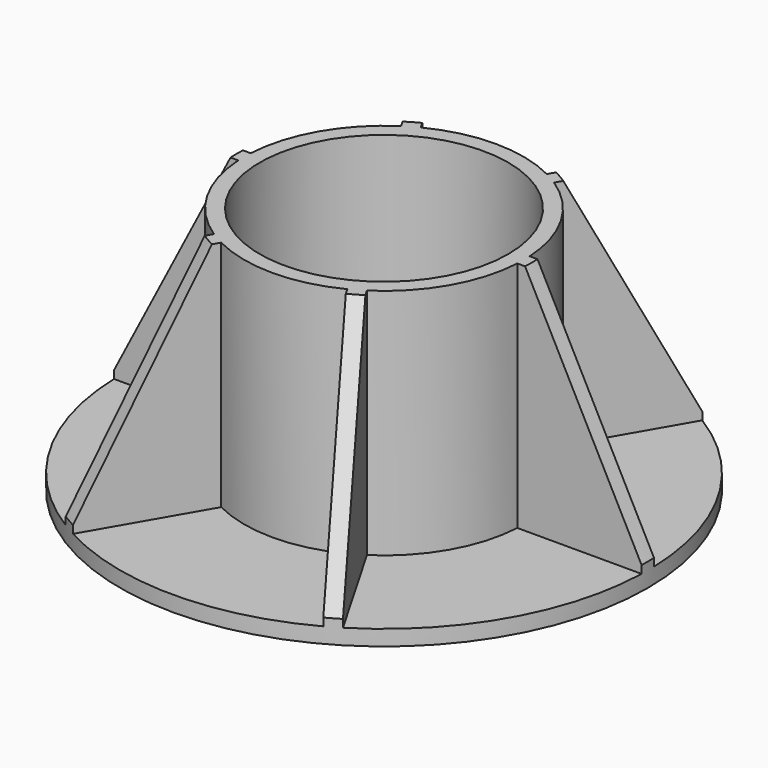
from build123d import *

# Parameters (mm, degrees)
F0_R            = 28.575
F0_R_2          = 25.4
F1_DEPTH        = 12.7
F2_R            = 53.975
F2_R_2          = 25.4
F3_DEPTH        = 50.8
F6_DEPTH        = 47.625
F6_COPIES_COUNT = 6


# Not quite as in the source:
# - a pattern or mirror of a feature is missing from the dataset's text; its kind, count and spacing are read off the source's solid


with BuildPart() as f1:
    # F0 (on Top) → F1 (new body)
    with BuildSketch(Plane.XY):
        Circle(F0_R)
        Circle(F0_R_2, mode=Mode.SUBTRACT)
    extrude(amount=F1_DEPTH)

    # F2 (on face) → F3 (join)
    with BuildSketch(Plane.XY.offset(12.7)):
        Circle(F2_R)
        Circle(F2_R_2, mode=Mode.SUBTRACT)
    extrude(amount=F3_DEPTH)

    # F5 (on face) → F6 (cut, through all)
    with BuildSketch(Plane.XY.offset(63.5)):
        with BuildLine():
            ThreePointArc((-15.6402496783, -23.9147070858), (-24.7466759131, -14.2875), (-28.5308686995, -1.5875))
            Line((-28.5308686995, -1.5875), (-53.9516493608, -1.5875))
            ThreePointArc((-53.9516493608, -1.5875), (-46.7437211693, -26.9875), (-28.3506400089, -45.9297489225))
            Line((-28.3506400089, -45.9297489225), (-15.6402496783, -23.9147070858))
        make_face()
    f6 = extrude(amount=-F6_DEPTH, mode=Mode.SUBTRACT)

    # F6_copies: F6 ×6 about axis
    f6_copies_axis = Axis((0, 0, 0), (0, 0, 1))
    for i in range(1, F6_COPIES_COUNT):
        add(f6.rotate(f6_copies_axis, i * 360 / F6_COPIES_COUNT), mode=Mode.SUBTRACT)

    # F7 (on Front) → F8 (revolve, cut)
    with BuildSketch(Plane.XZ):
        Polygon((-53.975, 17.4625), (-30.1625, 63.5), (-53.975, 63.5), align=None)
    revolve(axis=Axis((0, 0, 0), (0, 0, -1)), mode=Mode.SUBTRACT)


solid = f1.part
